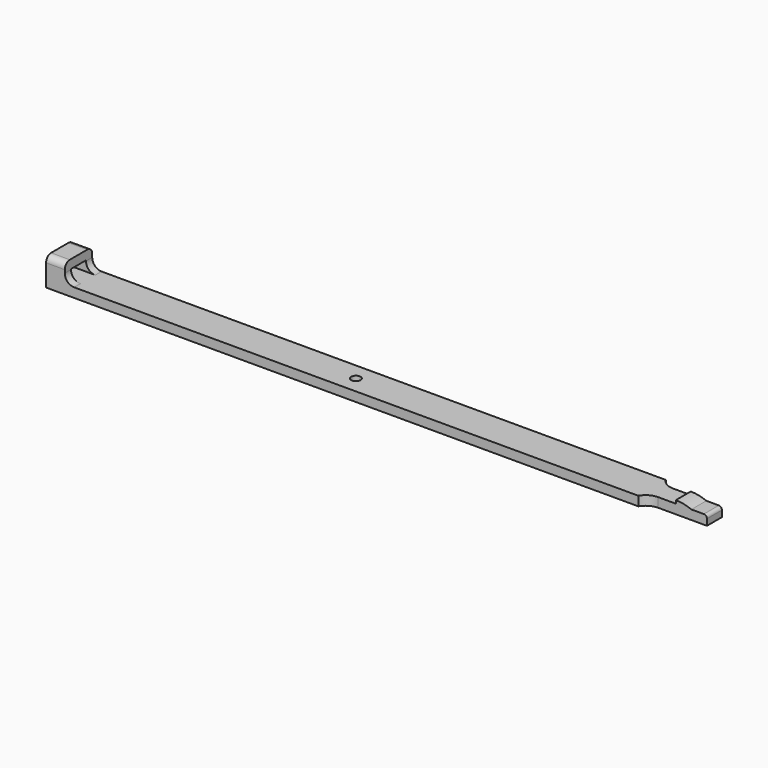
from build123d import *

# Parameters (mm, degrees)
F0_W         = 6
F0_H         = 11
F0_R         = 1.5
F1_DEPTH     = 3
F2_DEPTH     = 9
F3_W         = 6
F3_H         = 3.2
F4_DEPTH     = 15
F5_W         = 5
F5_H         = 6
F6_DEPTH     = 1
F7_T1_DEPTH  = 31
F8_R         = 3
F9_R         = 1
F10_T1_DEPTH = 3
F11_R        = 2


# Not quite as in the source:
# - a fillet or chamfer that OpenCascade refuses, or shapes differently, is made with other operations: its cross-section is extruded or revolved along the edge and cut away or added


with BuildPart() as f1:
    # F0 (on Top) → F1 (new body)
    with BuildSketch(Plane.XY):
        with Locations((-92, 0)):
            Rectangle(F0_W, F0_H)
        Polygon((-89, -5.5), (95, -5.5), (95, -3), (115, -3), (115, 3), (95, 3), (95, 5.5), (-89, 5.5), align=None)
        Circle(F0_R, mode=Mode.SUBTRACT)
    extrude(amount=F1_DEPTH)

    # F0 (on Top) → F2 (join)
    with BuildSketch(Plane.XY):
        with Locations((-92, 0)):
            Rectangle(F0_W, F0_H)
    extrude(amount=F2_DEPTH)

    # F3 (on face) → F4 (cut, symmetric)
    with BuildSketch(Plane(origin=(-95, 0, 0), x_dir=(0, -1, 0), z_dir=(-1, 0, 0))):
        with Locations((0, 4.6)):
            Rectangle(F3_W, F3_H)
    extrude(amount=F4_DEPTH, both=True, mode=Mode.SUBTRACT)

    # F5 (on face) → F6 (join)
    with BuildSketch(Plane.XY.offset(3)):
        with Locations((107.5, 0)):
            Rectangle(F5_W, F5_H)
    extrude(amount=F6_DEPTH)

    # F7: fillet of radius 13 on 1 edges, made by hand

    # F7_s2 → F7_t1 (cut)
    with BuildSketch(Plane.XZ.offset(-15.5)):
        with BuildLine():
            ThreePointArc((105, 4), (107.5495097568, 3.747548784), (110, 3))
            Line((110, 3), (110, 4))
            Line((110, 4), (105, 4))
        make_face()
    extrude(amount=F7_T1_DEPTH, mode=Mode.SUBTRACT)

    # F8
    f8_edges = [f1.edges().sort_by_distance(p)[0] for p in [
        (-89, -4.25, 3),
        (-89, 4.25, 3),
    ]]
    fillet(f8_edges, radius=F8_R)

    # F9
    f9_edges = [f1.edges().sort_by_distance(p)[0] for p in [
        (115, 0, 3),
    ]]
    fillet(f9_edges, radius=F9_R)

    # F10: fillet of radius 5 on 2 edges, made by hand

    # F10_s2 → F10_t1 (join)
    with BuildSketch(Plane.XY):
        with BuildLine():
            ThreePointArc((99.3301270189, -3), (96.8301270189, -3.6698729811), (95, -5.5))
            Line((95, -5.5), (95, -3))
            Line((95, -3), (99.3301270189, -3))
        make_face()
        with BuildLine():
            ThreePointArc((99.3301270189, 3), (96.8301270189, 3.6698729811), (95, 5.5))
            Line((95, 5.5), (95, 3))
            Line((95, 3), (99.3301270189, 3))
        make_face()
    extrude(amount=F10_T1_DEPTH)

    # F11
    f11_edges = [f1.edges().sort_by_distance(p)[0] for p in [
        (-92, 5.5, 9),
        (-92, -5.5, 9),
    ]]
    fillet(f11_edges, radius=F11_R)


solid = f1.part
